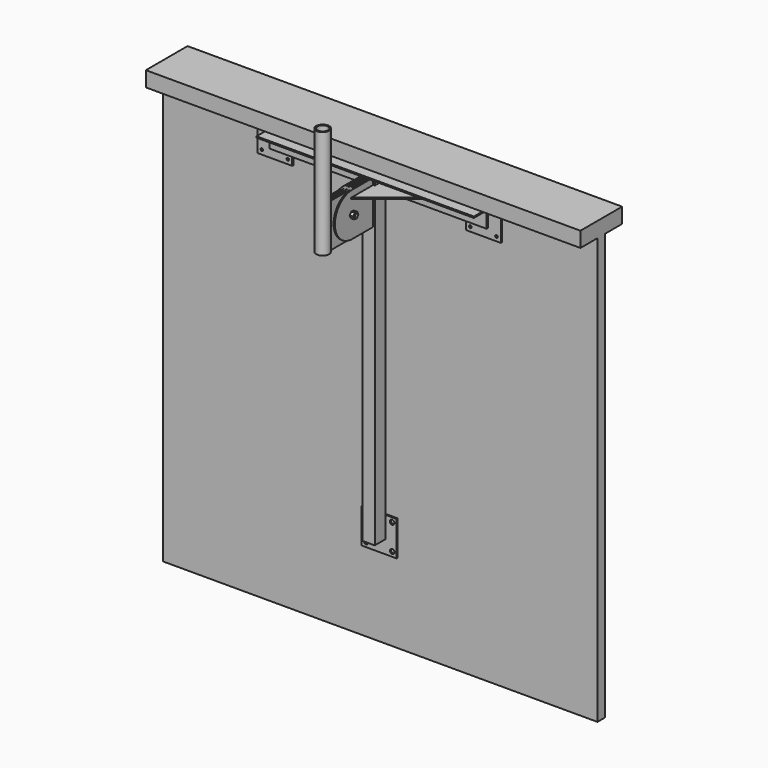
from build123d import *

# Parameters (mm, degrees)
F2_DEPTH       = 500
F3_W           = 80
F3_H           = 80
F3_R           = 3
F4_DEPTH       = 3
F3_R_2         = 5.2581355903
F6_DEPTH       = 250
F7_W           = 28.3992085606
F7_H           = 30.3552821279
F7_W_2         = 24.3992085606
F7_H_2         = 26.3552821279
F8_DEPTH       = 620
F8_DEPTH_BACK  = 123.8216329813
F9_W           = 3
F9_H           = 100
F10_DEPTH      = 110
F11_R          = 49.99999
F11_2_R        = 49.99999
F11_3_R        = 49.99999
F11_4_R        = 49.99999
F13_W          = 3
F13_H          = 100
F14_DEPTH      = 110
F15_R          = 49.99999
F15_2_R        = 49.99999
F15_3_R        = 49.99999
F16_R          = 4
F17_DEPTH      = 21
F18_R          = 15
F18_R_2        = 12
F19_DEPTH      = 150
F19_DEPTH_BACK = 100
F20_R          = 4
F21_DEPTH      = 30
F23_DEPTH      = 10
F25_DEPTH      = 8
F28_DEPTH      = 3


# Not quite as in the source:
# - a fillet or chamfer is up to 0.001 mm smaller than in the source, because OpenCascade refuses the exact size


with BuildPart() as f2:
    # F1 (on Right) → F2 (new body, symmetric)
    with BuildSketch(Plane.YZ):
        Polygon((11, 146.8216329813), (60, 146.8216329813), (60, 181.8216329813), (-60, 181.8216329813), (-60, 146.8216329813), (-11, 146.8216329813), (-11, -833.1783670187), (11, -833.1783670187), align=None)
    extrude(amount=F2_DEPTH, both=True)


with BuildPart() as f4:
    # F3 (on face) → F4 (new body)
    with BuildSketch(Plane.XZ.offset(11)):
        with Locations((-240, 106.8216329813)):
            Rectangle(F3_W, F3_H)
        with Locations((-270, 76.8216329813)):
            Circle(F3_R, mode=Mode.SUBTRACT)
        with Locations((-270, 136.8216329813)):
            Circle(F3_R, mode=Mode.SUBTRACT)
        with Locations((-210, 76.8216329813)):
            Circle(F3_R, mode=Mode.SUBTRACT)
        with Locations((-210, 136.8216329813)):
            Circle(F3_R, mode=Mode.SUBTRACT)
    extrude(amount=F4_DEPTH)


with BuildPart() as f4b:
    # F3 (on face) → F4, piece 2 (new body)
    with BuildSketch(Plane.XZ.offset(11)):
        with Locations((240, 106.8216329813)):
            Rectangle(F3_W, F3_H)
        with Locations((210, 76.8216329813)):
            Circle(F3_R, mode=Mode.SUBTRACT)
        with Locations((270, 76.8216329813)):
            Circle(F3_R, mode=Mode.SUBTRACT)
        with Locations((210, 136.8216329813)):
            Circle(F3_R, mode=Mode.SUBTRACT)
        with Locations((270, 136.8216329813)):
            Circle(F3_R, mode=Mode.SUBTRACT)
    extrude(amount=F4_DEPTH)


with BuildPart() as f4c:
    # F3 (on face) → F4, piece 3 (new body)
    with BuildSketch(Plane.XZ.offset(11)):
        with Locations((0, -610.3209847212)):
            Rectangle(F3_W, F3_H)
        with Locations((-30, -639.5133429766)):
            Circle(F3_R_2, mode=Mode.SUBTRACT)
        with Locations((-30, -580.3209847212)):
            Circle(F3_R_2, mode=Mode.SUBTRACT)
        with Locations((30, -639.5133429766)):
            Circle(F3_R_2, mode=Mode.SUBTRACT)
        with Locations((30, -580.3209847212)):
            Circle(F3_R_2, mode=Mode.SUBTRACT)
    extrude(amount=F4_DEPTH)


with BuildPart() as f6:
    # F5 (on Right) → F6 (new body, symmetric)
    with BuildSketch(Plane.YZ):
        Polygon((-14, 126.8216329813), (-54, 126.8216329813), (-54, 123.8216329813), (-17, 123.8216329813), (-17, 86.8216329813), (-14, 86.8216329813), align=None)
    extrude(amount=F6_DEPTH, both=True)


with BuildPart() as f8:
    # F7 (on Top) → F8 (new body, two sides)
    with BuildSketch(Plane.XY) as f8_sk:
        with Locations((0, -29.1776410639)):
            Rectangle(F7_W, F7_H)
        with Locations((0, -29.1776410639)):
            Rectangle(F7_W_2, F7_H_2, mode=Mode.SUBTRACT)
    extrude(amount=-F8_DEPTH)
    extrude(f8_sk.sketch, amount=F8_DEPTH_BACK)


with BuildPart() as f10:
    # F9 (on face) → F10 (new body)
    with BuildSketch(Plane.XZ.offset(44.3552821279)):
        with Locations((-3, 73.8216329813)):
            Rectangle(F9_W, F9_H)
    extrude(amount=F10_DEPTH)

    # F11 (radius 50 in the source; OpenCascade refuses exactly that, so slightly less here)
    f11_edges = [f10.edges().sort_by_distance(p)[0] for p in [
        (-3, -154.355282, 23.821633),
        (-3, -154.355282, 123.821633),
    ]]
    fillet(f11_edges, radius=F11_R)


with BuildPart() as f10b:
    # F9 (on face) → F10, piece 2 (new body)
    with BuildSketch(Plane.XZ.offset(44.3552821279)):
        with Locations((-9, 73.8216329813)):
            Rectangle(F9_W, F9_H)
    extrude(amount=F10_DEPTH)

    # F11#2 (radius 50 in the source; OpenCascade refuses exactly that, so slightly less here)
    f11_2_edges = [f10b.edges().sort_by_distance(p)[0] for p in [
        (-9, -154.355282, 23.821633),
        (-9, -154.355282, 123.821633),
    ]]
    fillet(f11_2_edges, radius=F11_2_R)


with BuildPart() as f10c:
    # F9 (on face) → F10, piece 3 (new body)
    with BuildSketch(Plane.XZ.offset(44.3552821279)):
        with Locations((3, 73.8216329813)):
            Rectangle(F9_W, F9_H)
    extrude(amount=F10_DEPTH)

    # F11#3 (radius 50 in the source; OpenCascade refuses exactly that, so slightly less here)
    f11_3_edges = [f10c.edges().sort_by_distance(p)[0] for p in [
        (3, -154.355282, 23.821633),
        (3, -154.355282, 123.821633),
    ]]
    fillet(f11_3_edges, radius=F11_3_R)


with BuildPart() as f10d:
    # F9 (on face) → F10, piece 4 (new body)
    with BuildSketch(Plane.XZ.offset(44.3552821279)):
        with Locations((9, 73.8216329813)):
            Rectangle(F9_W, F9_H)
    extrude(amount=F10_DEPTH)

    # F11#4 (radius 50 in the source; OpenCascade refuses exactly that, so slightly less here)
    f11_4_edges = [f10d.edges().sort_by_distance(p)[0] for p in [
        (9, -154.355282, 23.821633),
        (9, -154.355282, 123.821633),
    ]]
    fillet(f11_4_edges, radius=F11_4_R)


with BuildPart() as f14:
    # F13 (on offset) → F14 (new body)
    with BuildSketch(Plane.XZ.offset(164.3552821279)):
        with Locations((-6, 73.8216329813)):
            Rectangle(F13_W, F13_H)
    extrude(amount=-F14_DEPTH)

    # F15 (radius 50 in the source; OpenCascade refuses exactly that, so slightly less here)
    f15_edges = [f14.edges().sort_by_distance(p)[0] for p in [
        (-6, -54.355282, 123.821633),
        (-6, -54.355282, 23.821633),
    ]]
    fillet(f15_edges, radius=F15_R)


with BuildPart() as f14b:
    # F13 (on offset) → F14, piece 2 (new body)
    with BuildSketch(Plane.XZ.offset(164.3552821279)):
        with Locations((0, 73.8216329813)):
            Rectangle(F13_W, F13_H)
    extrude(amount=-F14_DEPTH)

    # F15#2 (radius 50 in the source; OpenCascade refuses exactly that, so slightly less here)
    f15_2_edges = [f14b.edges().sort_by_distance(p)[0] for p in [
        (0, -54.355282, 123.821633),
        (0, -54.355282, 23.821633),
    ]]
    fillet(f15_2_edges, radius=F15_2_R)


with BuildPart() as f14c:
    # F13 (on offset) → F14, piece 3 (new body)
    with BuildSketch(Plane.XZ.offset(164.3552821279)):
        with Locations((6, 73.8216329813)):
            Rectangle(F13_W, F13_H)
    extrude(amount=-F14_DEPTH)

    # F15#3 (radius 50 in the source; OpenCascade refuses exactly that, so slightly less here)
    f15_3_edges = [f14c.edges().sort_by_distance(p)[0] for p in [
        (6, -54.355282, 123.821633),
        (6, -54.355282, 23.821633),
    ]]
    fillet(f15_3_edges, radius=F15_3_R)


with BuildPart() as f17_tool:
    # F16 (on face) → F17 (new body, through all)
    with BuildSketch(Plane(origin=(-10.5, 0, 0), x_dir=(0, -1, 0), z_dir=(-1, 0, 0))):
        with Locations((104.3552821279, 73.8216329813)):
            Circle(F16_R)
    extrude(amount=-F17_DEPTH)


with BuildPart() as f10_1:
    add(f10.part)

    # F17: cut by f17_tool
    add(f17_tool.part, mode=Mode.SUBTRACT)


with BuildPart() as f10b_1:
    add(f10b.part)

    # F17: cut by f17_tool
    add(f17_tool.part, mode=Mode.SUBTRACT)


with BuildPart() as f10c_1:
    add(f10c.part)

    # F17: cut by f17_tool
    add(f17_tool.part, mode=Mode.SUBTRACT)


with BuildPart() as f10d_1:
    add(f10d.part)

    # F17: cut by f17_tool
    add(f17_tool.part, mode=Mode.SUBTRACT)


with BuildPart() as f14_1:
    add(f14.part)

    # F17: cut by f17_tool
    add(f17_tool.part, mode=Mode.SUBTRACT)


with BuildPart() as f14b_1:
    add(f14b.part)

    # F17: cut by f17_tool
    add(f17_tool.part, mode=Mode.SUBTRACT)


with BuildPart() as f14c_1:
    add(f14c.part)

    # F17: cut by f17_tool
    add(f17_tool.part, mode=Mode.SUBTRACT)


with BuildPart() as f19:
    # F18 (on face) → F19 (new body, two sides)
    with BuildSketch(Plane.XY.offset(123.8216329813)) as f19_sk:
        with Locations((0, -176.3552821279)):
            Circle(F18_R)
        with Locations((0, -176.3552821279)):
            Circle(F18_R_2, mode=Mode.SUBTRACT)
    extrude(amount=F19_DEPTH)
    extrude(f19_sk.sketch, amount=-F19_DEPTH_BACK)


with BuildPart() as f21:
    # F20 (on face) → F21 (new body)
    with BuildSketch(Plane(origin=(-10.5, 0, 0), x_dir=(0, -1, 0), z_dir=(-1, 0, 0))):
        with Locations((104.3552821279, 73.8216329813)):
            Circle(F20_R)
    extrude(amount=-F21_DEPTH)

    # F22 (on face) → F23 (join)
    with BuildSketch(Plane(origin=(-10.5, 0, 0), x_dir=(0, -1, 0), z_dir=(-1, 0, 0))):
        Polygon((107.8366015876, 67.1722910475), (111.8544408908, 73.5118731053), (108.3731214311, 80.161215039), (100.8739626681, 80.4709749151), (96.8561233649, 74.1313928573), (100.3374428246, 67.4820509236), align=None)
    extrude(amount=F23_DEPTH)


with BuildPart() as f25:
    # F24 (on face) → F25 (new body)
    with BuildSketch(Plane.YZ.offset(10.5)):
        Polygon((-101.4925720239, 66.8834614503), (-96.9152942742, 72.8317268895), (-99.7780043781, 79.7698984206), (-107.2179922318, 80.7598045124), (-111.7952699815, 74.8115390732), (-108.9325598776, 67.8733675421), align=None)
    extrude(amount=F25_DEPTH)


with BuildPart() as f28:
    # F27 (on offset) → F28 (new body)
    with BuildSketch(Plane(origin=(0, 0, 108.8216329813), x_dir=(1, 0, 0), z_dir=(0, 0, -1))):
        Polygon((121.1775859371, 17), (10.5, 107.7398955822), (10.5, 44.3552821279), (14.1996042803, 44.3552821279), (14.1996042803, 17), align=None)
    extrude(amount=F28_DEPTH)


solid = Compound([f2.part, f4.part, f4b.part, f4c.part, f6.part, f8.part, f10_1.part, f10b_1.part, f10c_1.part, f10d_1.part, f14_1.part, f14b_1.part, f14c_1.part, f19.part, f21.part, f25.part, f28.part])
